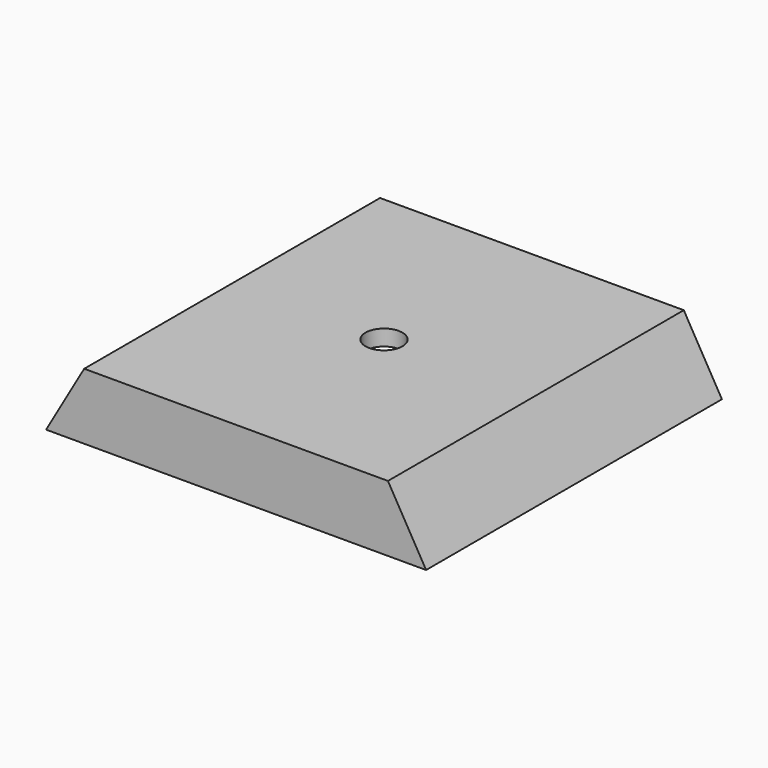
from build123d import *

# Parameters (mm, degrees)
F0_W        = 46.0375
F0_H        = 44.45
F1_DEPTH    = 7.9375
F2_T1_DEPTH = 87.1311818198
F3_T        = -1.905
F5_D        = 4.445


# Not quite as in the source:
# - a fillet or chamfer that OpenCascade refuses, or shapes differently, is made with other operations: its cross-section is extruded or revolved along the edge and cut away or added


with BuildPart() as f1:
    # F0 (on Top) → F1 (new body)
    with BuildSketch(Plane.XY):
        with Locations((3.8099996746, 17.1172746531)):
            Rectangle(F0_W, F0_H)
    extrude(amount=F1_DEPTH)

    # F2: chamfer of 4.7625 x 8.248891971 on 2 edges, made by hand

    # F2_s2 → F2_t1 (cut)
    with BuildSketch(Plane.XZ.offset(-60.682865563)):
        Polygon((-19.2087503254, -0.311391971), (-14.4462503254, 7.9375), (-19.2087503254, 7.9375), align=None)
        Polygon((26.8287496746, -0.311391971), (22.0662496746, 7.9375), (26.8287496746, 7.9375), align=None)
    extrude(amount=F2_T1_DEPTH, mode=Mode.SUBTRACT)

    # F3
    f3_openings = [f1.faces().sort_by_distance(p)[0] for p in [
        (3.81, 17.117275, 0),
    ]]
    offset(amount=F3_T, openings=f3_openings)

    # F5 (through all)
    with Locations(Plane.XY.offset(7.9375)):
        with Locations((3.8099996746, 17.1172746531)):
            Hole(F5_D / 2)


solid = f1.part
